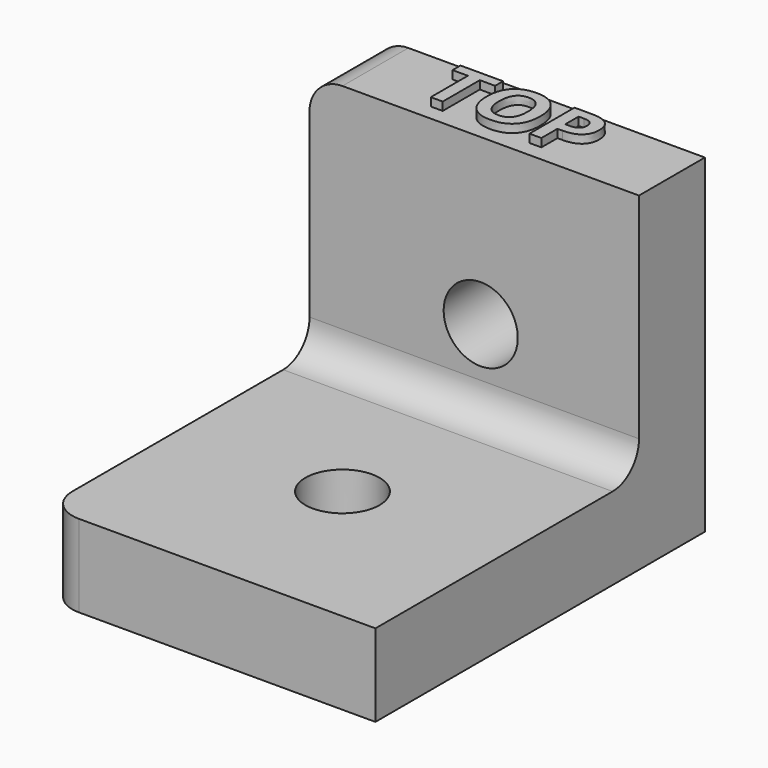
from build123d import *

# Parameters (mm, degrees)
F0_W         = 20
F0_H         = 20
F0_R         = 2.25
F1_DEPTH     = 5
F0_H_2       = 5
F2_DEPTH     = 20
F3_R         = 2
F4_R         = 2.2512233174
F5_DEPTH     = 6
F6_TEXT_SIZE = 4.7885838689
F7_DEPTH     = 0.5


# Not quite as in the source:
# - Text() gives the source's letters only with a copy of the font that has no kerning and outlines rounded to 1/6400 em; it was checked with that copy


with BuildPart() as f1:
    # F0 (on Top) → F1 (new body)
    with BuildSketch(Plane.XY):
        with Locations((0.34482753, 10)):
            Rectangle(F0_W, F0_H)
        with Locations((0.34482753, 10)):
            Circle(F0_R, mode=Mode.SUBTRACT)
    extrude(amount=F1_DEPTH)

    # F0 (on Top) → F2 (join)
    with BuildSketch(Plane.XY):
        with Locations((0.34482753, 22.5)):
            Rectangle(F0_W, F0_H_2)
    extrude(amount=F2_DEPTH)

    # F3
    f3_edges = [f1.edges().sort_by_distance(p)[0] for p in [
        (-9.655172, 22.5, 20),
        (-9.655172, 0, 2.5),
        (0.344828, 20, 5),
    ]]
    fillet(f3_edges, radius=F3_R)

    # F4 (on face) → F5 (cut)
    with BuildSketch(Plane(origin=(0, 25, 0), x_dir=(-1, 0, 0), z_dir=(0, 1, 0))):
        with Locations((-0.7373829139, 10)):
            Circle(F4_R)
    extrude(amount=-F5_DEPTH, mode=Mode.SUBTRACT)

    # F6 (on face) → F7 (join)
    with BuildSketch(Plane.XY.offset(20)):
        with Locations((-4.0949350223, 20.9690146148)):
            Text('TOP', F6_TEXT_SIZE, font='Open Sans', font_style=FontStyle.BOLD, text_align=(TextAlign.LEFT, TextAlign.BOTTOM))
    extrude(amount=F7_DEPTH)


solid = f1.part
